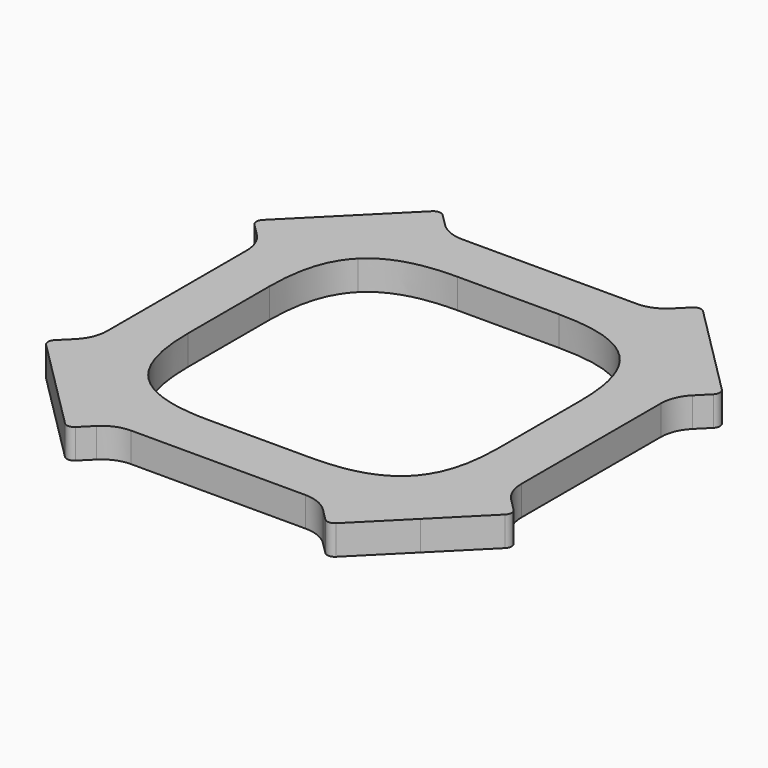
from build123d import *

# Parameters (mm, degrees)
F1_DEPTH = 4


# Not quite as in the source:
# - a feature names something its author has since deleted; it is built from what else it names


with BuildPart() as f1:
    # F0 (on Top) → F1 (new body)
    with BuildSketch(Plane.XY):
        Polygon((-108.5178543984, -51.6479864335), (-108.5178543984, -37.9322576809), (-115.5178543984, -30.9322576809), (-115.5178543984, -33.0033254928), (-115.5178543984, -56.5769186216), (-115.5178543984, -58.6479864335), align=None)
        with BuildLine():
            Line((-115.5178543984, -33.0033254928), (-115.5178543984, -30.9322576809))
            Line((-115.5178543984, -30.9322576809), (-116.982320508, -29.4677915713))
            ThreePointArc((-116.982320508, -29.4677915713), (-115.89845674, -31.0899083208), (-115.5178543984, -33.0033254928))
        make_face()
        with BuildLine():
            Line((-58.0533882883, -29.4677915708), (-59.5178543984, -30.9322576809))
            Line((-59.5178543984, -30.9322576809), (-59.5178543984, -33.0033254928))
            ThreePointArc((-59.5178543984, -33.0033254928), (-59.1372520566, -31.0899083205), (-58.0533882883, -29.4677915708))
        make_face()
        Polygon((-66.5178543984, -37.9322576809), (-66.5178543984, -51.6479864335), (-59.5178543984, -58.6479864335), (-59.5178543984, -56.5769186216), (-59.5178543984, -33.0033254928), (-59.5178543984, -30.9322576809), align=None)
        with BuildLine():
            Line((-59.5178543984, -56.5769186216), (-59.5178543984, -58.6479864335))
            Line((-59.5178543984, -58.6479864335), (-58.0533883237, -60.1124525081))
            ThreePointArc((-58.0533883237, -60.1124525081), (-59.1372520662, -58.4903357707), (-59.5178543984, -56.5769186216))
        make_face()
        with BuildLine():
            Line((-116.982320508, -60.1124525431), (-115.5178543984, -58.6479864335))
            Line((-115.5178543984, -58.6479864335), (-115.5178543984, -56.5769186216))
            ThreePointArc((-115.5178543984, -56.5769186216), (-115.89845674, -58.4903357936), (-116.982320508, -60.1124525431))
        make_face()
        Polygon((-101.3757187746, -16.7901220572), (-94.3757187746, -23.7901220572), (-80.6599900221, -23.7901220572), (-73.6599900221, -16.7901220572), (-75.731057834, -16.7901220572), (-99.3046509628, -16.7901220572), align=None)
        with BuildLine():
            Line((-102.8401848842, -15.3256559476), (-101.3757187746, -16.7901220572))
            Line((-101.3757187746, -16.7901220572), (-99.3046509628, -16.7901220572))
            ThreePointArc((-99.3046509628, -16.7901220572), (-101.2180681347, -16.4095197156), (-102.8401848842, -15.3256559476))
        make_face()
        with BuildLine():
            Line((-75.731057834, -16.7901220572), (-73.6599900221, -16.7901220572))
            Line((-73.6599900221, -16.7901220572), (-72.1955238561, -15.3256558912))
            ThreePointArc((-72.1955238561, -15.3256558912), (-73.8176406251, -16.4095197003), (-75.731057834, -16.7901220572))
        make_face()
        Polygon((-73.6599900221, -72.7901220572), (-80.6599900221, -65.7901220572), (-94.3757187746, -65.7901220572), (-101.3757187746, -72.7901220572), (-99.3046509628, -72.7901220572), (-75.731057834, -72.7901220572), align=None)
        with BuildLine():
            Line((-99.3046509628, -72.7901220572), (-101.3757187746, -72.7901220572))
            Line((-101.3757187746, -72.7901220572), (-102.8401848842, -74.2545881668))
            ThreePointArc((-102.8401848842, -74.2545881668), (-101.2180681347, -73.1707243988), (-99.3046509628, -72.7901220572))
        make_face()
        with BuildLine():
            Line((-72.1955239691, -74.2545881102), (-73.6599900221, -72.7901220572))
            Line((-73.6599900221, -72.7901220572), (-75.731057834, -72.7901220572))
            ThreePointArc((-75.731057834, -72.7901220572), (-73.8176406989, -73.1707243835), (-72.1955239691, -74.2545881102))
        make_face()
        with BuildLine():
            Line((-105.1967865865, -27.1111898691), (-112.1958810618, -20.1120953938))
            Line((-112.1958810618, -20.1120953938), (-118.5598420925, -26.4760564245))
            ThreePointArc((-118.5598420925, -26.4760564245), (-118.8527353113, -27.1831632057), (-118.5598420925, -27.8902699868))
            Line((-118.5598420925, -27.8902699868), (-116.982320508, -29.4677915713))
            Line((-116.982320508, -29.4677915713), (-115.5178543984, -30.9322576809))
            Line((-115.5178543984, -30.9322576809), (-108.5178543984, -37.9322576809))
            add(Edge.make_bspline(
                [(-108.5178543984, -37.9322576809), (-108.5178543984, -32.9322576809), (-107.4823204924, -29.396723775), (-105.1967865865, -27.1111898691)],
                knots=[0, 0, 0, 0, 10, 10, 10, 10], degree=3))
        make_face()
        with BuildLine():
            Line((-105.8319200311, -13.7481343631), (-112.1958810618, -20.1120953938))
            Line((-112.1958810618, -20.1120953938), (-105.1967865865, -27.1111898691))
            add(Edge.make_bspline(
                [(-105.1967865865, -27.1111898691), (-102.9112526806, -24.8256559631), (-99.3757187746, -23.7901220572), (-94.3757187746, -23.7901220572)],
                knots=[10, 10, 10, 10, 20, 20, 20, 20], degree=3))
            Line((-94.3757187746, -23.7901220572), (-101.3757187746, -16.7901220572))
            Line((-101.3757187746, -16.7901220572), (-102.8401848842, -15.3256559476))
            Line((-102.8401848842, -15.3256559476), (-104.4177064687, -13.7481343631))
            ThreePointArc((-104.4177064687, -13.7481343631), (-105.1248132499, -13.4552411443), (-105.8319200311, -13.7481343631))
        make_face()
        with BuildLine():
            Line((-73.6599900221, -16.7901220572), (-80.6599900221, -23.7901220572))
            add(Edge.make_bspline(
                [(-80.6599900221, -23.7901220572), (-75.6599900221, -23.7901220572), (-72.1244561162, -24.8256559631), (-69.8389222102, -27.1111898691)],
                knots=[0, 0, 0, 0, 10, 10, 10, 10], degree=3))
            Line((-69.8389222102, -27.1111898691), (-62.839827735, -20.1120953938))
            Line((-62.839827735, -20.1120953938), (-69.2037887656, -13.7481343631))
            ThreePointArc((-69.2037887656, -13.7481343631), (-69.9108955468, -13.4552411443), (-70.618002328, -13.7481343631))
            Line((-70.618002328, -13.7481343631), (-72.1955238561, -15.3256558912))
            Line((-72.1955238561, -15.3256558912), (-73.6599900221, -16.7901220572))
        make_face()
        with BuildLine():
            Line((-62.839827735, -20.1120953938), (-69.8389222102, -27.1111898691))
            add(Edge.make_bspline(
                [(-69.8389222102, -27.1111898691), (-67.5533883043, -29.396723775), (-66.5178543984, -32.9322576809), (-66.5178543984, -37.9322576809)],
                knots=[10, 10, 10, 10, 20, 20, 20, 20], degree=3))
            Line((-66.5178543984, -37.9322576809), (-59.5178543984, -30.9322576809))
            Line((-59.5178543984, -30.9322576809), (-58.0533882883, -29.4677915708))
            Line((-58.0533882883, -29.4677915708), (-56.4758667043, -27.8902699868))
            ThreePointArc((-56.4758667043, -27.8902699868), (-56.1829734855, -27.1831632057), (-56.4758667043, -26.4760564245))
            Line((-56.4758667043, -26.4760564245), (-62.839827735, -20.1120953938))
        make_face()
        with BuildLine():
            add(Edge.make_bspline(
                [(-69.8389222102, -62.4690542453), (-67.5533883043, -60.1835203394), (-66.5178543984, -56.6479864335), (-66.5178543984, -51.6479864335)],
                knots=[10, 10, 10, 10, 20, 20, 20, 20], degree=3))
            Line((-69.8389222102, -62.4690542453), (-62.839827735, -69.4681487206))
            Line((-62.839827735, -69.4681487206), (-56.4758667043, -63.1041876899))
            ThreePointArc((-56.4758667043, -63.1041876899), (-56.1829734855, -62.3970809087), (-56.4758667043, -61.6899741276))
            Line((-56.4758667043, -61.6899741276), (-58.0533883237, -60.1124525081))
            Line((-58.0533883237, -60.1124525081), (-59.5178543984, -58.6479864335))
            Line((-59.5178543984, -58.6479864335), (-66.5178543984, -51.6479864335))
        make_face()
        with BuildLine():
            Line((-62.839827735, -69.4681487206), (-69.8389222102, -62.4690542453))
            add(Edge.make_bspline(
                [(-80.6599900221, -65.7901220572), (-75.6599900221, -65.7901220572), (-72.1244561162, -64.7545881513), (-69.8389222102, -62.4690542453)],
                knots=[0, 0, 0, 0, 10, 10, 10, 10], degree=3))
            Line((-80.6599900221, -65.7901220572), (-73.6599900221, -72.7901220572))
            Line((-73.6599900221, -72.7901220572), (-72.1955239691, -74.2545881102))
            Line((-72.1955239691, -74.2545881102), (-70.618002328, -75.8321097513))
            ThreePointArc((-70.618002328, -75.8321097513), (-69.9108955468, -76.1250029701), (-69.2037887656, -75.8321097513))
            Line((-69.2037887656, -75.8321097513), (-62.839827735, -69.4681487206))
        make_face()
        with BuildLine():
            add(Edge.make_bspline(
                [(-105.1967865865, -62.4690542453), (-102.9112526806, -64.7545881513), (-99.3757187746, -65.7901220572), (-94.3757187746, -65.7901220572)],
                knots=[10, 10, 10, 10, 20, 20, 20, 20], degree=3))
            Line((-105.1967865865, -62.4690542453), (-112.1958810618, -69.4681487206))
            Line((-112.1958810618, -69.4681487206), (-105.8319200311, -75.8321097513))
            ThreePointArc((-105.8319200311, -75.8321097513), (-105.1248132499, -76.1250029701), (-104.4177064687, -75.8321097513))
            Line((-104.4177064687, -75.8321097513), (-102.8401848842, -74.2545881668))
            Line((-102.8401848842, -74.2545881668), (-101.3757187746, -72.7901220572))
            Line((-101.3757187746, -72.7901220572), (-94.3757187746, -65.7901220572))
        make_face()
        with BuildLine():
            add(Edge.make_bspline(
                [(-108.5178543984, -51.6479864335), (-108.5178543984, -56.6479864335), (-107.4823204924, -60.1835203394), (-105.1967865865, -62.4690542453)],
                knots=[0, 0, 0, 0, 10, 10, 10, 10], degree=3))
            Line((-108.5178543984, -51.6479864335), (-115.5178543984, -58.6479864335))
            Line((-115.5178543984, -58.6479864335), (-116.982320508, -60.1124525431))
            Line((-116.982320508, -60.1124525431), (-118.5598420925, -61.6899741276))
            ThreePointArc((-118.5598420925, -61.6899741276), (-118.8527353113, -62.3970809087), (-118.5598420925, -63.1041876899))
            Line((-118.5598420925, -63.1041876899), (-112.1958810618, -69.4681487206))
            Line((-112.1958810618, -69.4681487206), (-105.1967865865, -62.4690542453))
        make_face()
    extrude(amount=F1_DEPTH)


solid = f1.part
